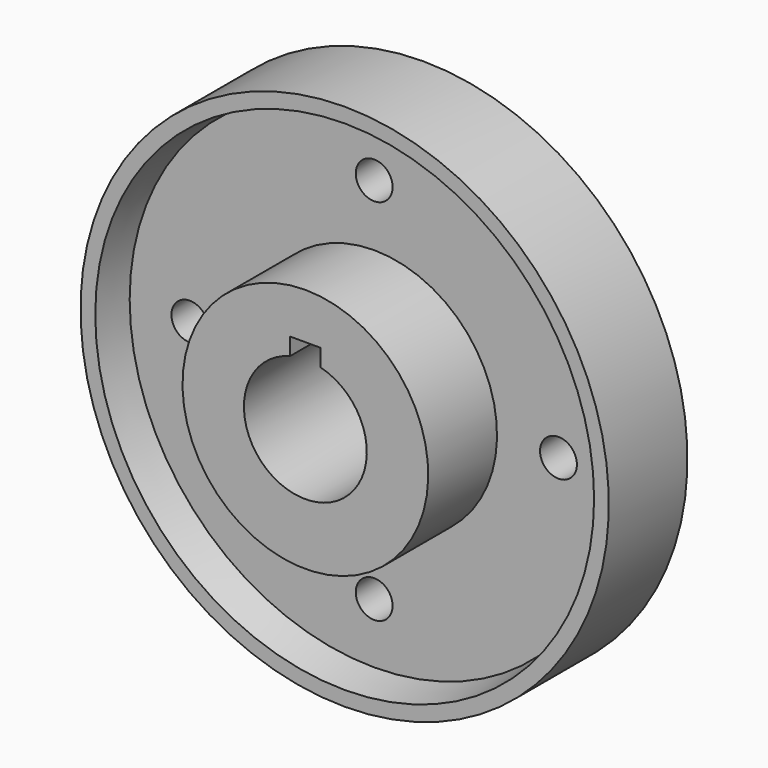
from build123d import *

# Parameters (mm, degrees)
F2_R     = 30
F2_R_2   = 15
F3_DEPTH = 2
F4_SIZE  = 1.99999
F5_R     = 4.5
F6_DEPTH = 25
F7_COUNT = 4
F8_W     = 7.5
F8_H     = 7.5
F9_DEPTH = 50


# Not quite as in the source:
# - a fillet or chamfer is up to 0.001 mm smaller than in the source, because OpenCascade refuses the exact size


with BuildPart() as f1:
    # F0 (on Right) → F1 (revolve)
    with BuildSketch(Plane.YZ):
        Polygon((0, 15), (0, 64.5), (-24, 64.5), (-24, 60.9), (-15, 59.7), (-15, 30), (-36, 30), (-36, 15), align=None)
    revolve(axis=Axis((0, -28.2661654055, 0), (0, -1, 0)))

    # F2 (on face) → F3 (join)
    with BuildSketch(Plane(origin=(0, 0, 0), x_dir=(-1, 0, 0), z_dir=(0, 1, 0))):
        Circle(F2_R)
        Circle(F2_R_2, mode=Mode.SUBTRACT)
    extrude(amount=F3_DEPTH)

    # F4 (size 2 in the source; OpenCascade refuses exactly that, so slightly less here)
    f4_edges = [f1.edges().sort_by_distance(p)[0] for p in [
        (30, 2, 0),
    ]]
    chamfer(f4_edges, length=F4_SIZE)

    # F5 (on face) → F6 (cut)
    with BuildSketch(Plane(origin=(0, 0, 0), x_dir=(-1, 0, 0), z_dir=(0, 1, 0))):
        with Locations((0, 45)):
            Circle(F5_R)
    f6 = extrude(amount=-F6_DEPTH, mode=Mode.SUBTRACT)

    # F7: F6 ×4 about axis
    f7_axis = Axis((0, 2, 0), (0, 1, 0))
    for i in range(1, F7_COUNT):
        add(f6.rotate(f7_axis, i * 360 / F7_COUNT), mode=Mode.SUBTRACT)

    # F8 (on face) → F9 (cut)
    with BuildSketch(Plane(origin=(0, 2, 0), x_dir=(-1, 0, 0), z_dir=(0, 1, 0))):
        with Locations((0, 15)):
            Rectangle(F8_W, F8_H)
    extrude(amount=-F9_DEPTH, mode=Mode.SUBTRACT)


solid = f1.part
